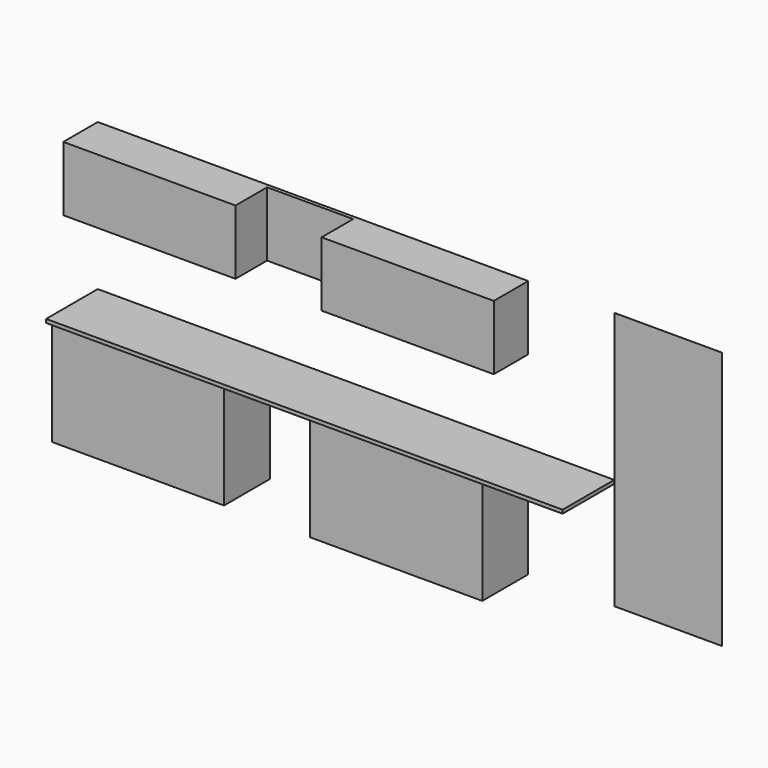
from build123d import *

# Parameters (mm, degrees)
F0_W     = 609.6
F0_H     = 762
F1_DEPTH = 406.4
F2_DEPTH = 0.254
F0_H_2   = 457.2
F3_DEPTH = 304.8
F4_W     = 1219.2
F4_H     = 406.4
F5_DEPTH = 25.4
F6_DEPTH = 25.4


with BuildPart() as f1:
    # F0 (on Front) → F1 (new body)
    with BuildSketch(Plane.XZ):
        with Locations((609.6, 0)):
            Rectangle(F0_W, F0_H)
        Rectangle(F0_W, F0_H)
    extrude(amount=F1_DEPTH)



with BuildPart() as f1b:
    # F0 (on Front) → F1, piece 2 (new body)
    with BuildSketch(Plane.XZ):
        with Locations((-1828.8, 0)):
            Rectangle(F0_W, F0_H)
        with Locations((-1219.2, 0)):
            Rectangle(F0_W, F0_H)
    extrude(amount=F1_DEPTH)


with BuildPart() as f2:
    # F0 (on Front) → F2 (new body)
    with BuildSketch(Plane.XZ):
        Polygon((1524, 381), (1524, -381), (2286, -381), (2286, 1447.8), (1524, 1447.8), (1524, 990.6), align=None)
    extrude(amount=F2_DEPTH)


with BuildPart() as f3:
    # F0 (on Front) → F3 (new body)
    with BuildSketch(Plane.XZ):
        with Locations((-1219.2, 1219.2)):
            Rectangle(F0_W, F0_H_2)
        with Locations((-1828.8, 1219.2)):
            Rectangle(F0_W, F0_H_2)
    extrude(amount=F3_DEPTH)



with BuildPart() as f3b:
    # F0 (on Front) → F3, piece 2 (new body)
    with BuildSketch(Plane.XZ):
        with Locations((609.6, 1219.2)):
            Rectangle(F0_W, F0_H_2)
        with Locations((0, 1219.2)):
            Rectangle(F0_W, F0_H_2)
    extrude(amount=F3_DEPTH)


with BuildPart() as f1_1:
    add(f1.part)

    add(f1b.part)  # F5 merges F1b
    # F4 (on face) → F5 (join)
    with BuildSketch(Plane.XY.offset(381)):
        Polygon((1523.5787630081, -457.2), (1523.5787630081, 0), (-914.4, 0), (-914.4, -406.4), (-2133.6, -406.4), (-2133.6, -457.2), align=None)
        with Locations((-1524, -203.2)):
            Rectangle(F4_W, F4_H)
    extrude(amount=F5_DEPTH)


with BuildPart() as f3_1:
    add(f3.part)

    add(f3b.part)  # F6 merges F3b
    # F0 (on Front) → F6 (join)
    with BuildSketch(Plane.XZ):
        with Locations((0, 1219.2)):
            Rectangle(F0_W, F0_H_2)
        with Locations((-609.6, 1219.2)):
            Rectangle(F0_W, F0_H_2)
    extrude(amount=F6_DEPTH)


solid = Compound([f2.part, f1_1.part, f3_1.part])
